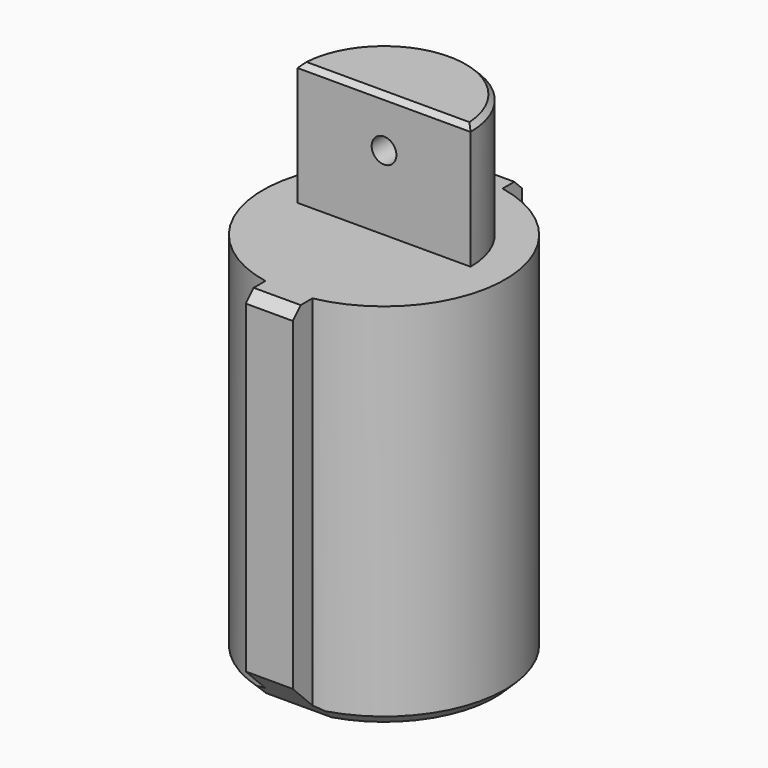
from build123d import *

# Parameters (mm, degrees)
F1_R          = 4.9
F2_DEPTH      = 5
F2_DEPTH_BACK = 15
F5_W          = 1.9
F5_H          = 15
F3_R          = 4.9
F7_DEPTH      = 5.001
F8_R          = 0.5
F9_DEPTH      = 5.801
F10_SIZE      = 0.2
F11_SIZE      = 0.4
F12_T1_DEPTH  = 9.6150489639
F13_SIZE      = 0.4


# Not quite as in the source:
# - a fillet or chamfer that OpenCascade refuses, or shapes differently, is made with other operations: its cross-section is extruded or revolved along the edge and cut away or added
# - a pattern or mirror of a feature is missing from the dataset's text; its kind, count and spacing are read off the source's solid


with BuildPart() as f2:
    # F1 (on Top) → F2 (new body, two sides)
    with BuildSketch(Plane.XY) as f2_sk:
        Circle(F1_R)
    extrude(amount=F2_DEPTH)
    extrude(f2_sk.sketch, amount=-F2_DEPTH_BACK)

    # F5 (on offset) → F6 (join, up to the next surface of F2)
    with BuildSketch(Plane.XZ.offset(-5.8)):
        with Locations((0, -7.5)):
            Rectangle(F5_W, F5_H)
    f6 = extrude(until=Until.NEXT)

    # F6_copies: F6 across plane
    add(f6.mirror(Plane(origin=(0, 0, 0), x_dir=(0, 0, -1), z_dir=(0, -1, 0))))

    # F3 (on Top) → F7 (cut, through all)
    with BuildSketch(Plane.XY):
        Circle(F3_R)
        with BuildLine():
            ThreePointArc((-3.5, 0), (0, 3.5), (3.5, 0))
            Line((3.5, 0), (-3.5, 0))
        make_face(mode=Mode.SUBTRACT)
    extrude(amount=F7_DEPTH, mode=Mode.SUBTRACT)

    # F8 (on face) → F9 (cut, through all)
    with BuildSketch(Plane.XZ):
        with Locations((0, 3)):
            Circle(F8_R)
    extrude(amount=-F9_DEPTH, mode=Mode.SUBTRACT)

    # F10
    f10_edges = [f2.edges().sort_by_distance(p)[0] for p in [
        (0, 3.5, 5),
        (0, 0, 5),
    ]]
    chamfer(f10_edges, length=F10_SIZE)

    # F11
    f11_edges = [f2.edges().sort_by_distance(p)[0] for p in [
        (-4.9, 0, -15),
    ]]
    chamfer(f11_edges, length=F11_SIZE)

    # F12: chamfer of 1.5 on 2 edges, made by hand

    # F12_s2 → F12_t1 (cut)
    with BuildSketch(Plane.YZ.offset(-4.8075244819)):
        Polygon((4.3, -15), (5.8, -13.5), (5.8, -15), align=None)
        Polygon((-4.3, -15), (-5.8, -13.5), (-5.8, -15), align=None)
    extrude(amount=F12_T1_DEPTH, mode=Mode.SUBTRACT)

    # F13
    f13_edges = [f2.edges().sort_by_distance(p)[0] for p in [
        (0, 5.8, 0),
        (0, -5.8, 0),
        (4.9, 0, -15),
    ]]
    chamfer(f13_edges, length=F13_SIZE)


solid = f2.part
